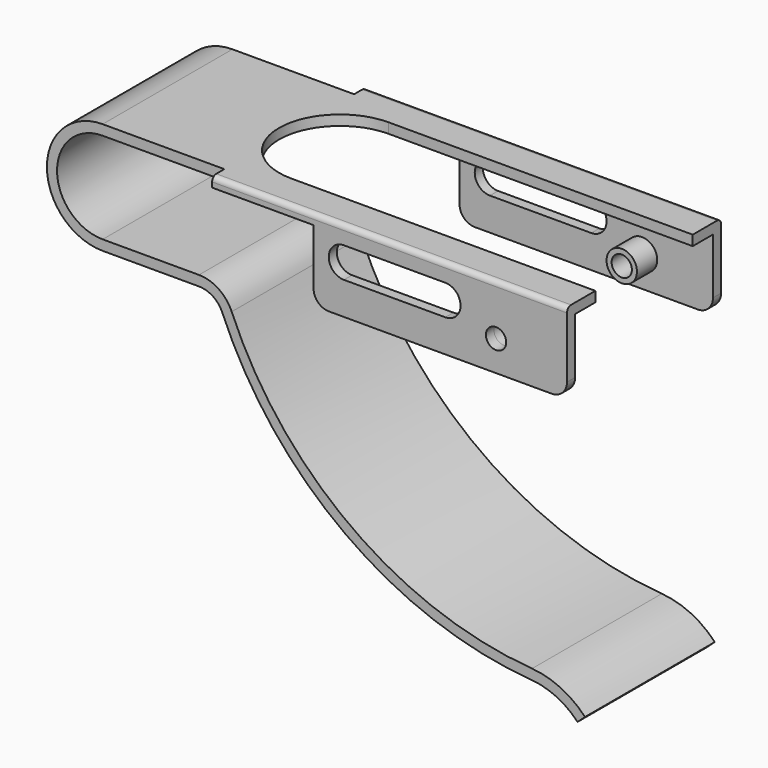
from build123d import *

# Parameters (mm, degrees)
F1_DEPTH  = 16
F2_W      = 70
F2_H      = 3
F3_DEPTH  = 2
F4_W      = 50
F4_H      = 14
F5_DEPTH  = 2
F6_R      = 1
F9_DEPTH  = 2
F11_DEPTH = 38.001
F13_D     = 4
F14_R     = 3
F14_R_2   = 2
F15_DEPTH = 5
F16_R     = 3


# Not quite as in the source:
# - a pattern or mirror of a feature is missing from the dataset's text; its kind, count and spacing are read off the source's solid


with BuildPart() as f1:
    # F0 (on Front) → F1 (new body)
    with BuildSketch(Plane.XZ):
        with BuildLine():
            Line((94, 11), (0, 11))
            ThreePointArc((0, 11), (-11, 0), (0, -11))
            Line((0, -11), (19, -11))
            ThreePointArc((19, -11), (21.7681124643, -11.8361612201), (23.6103896104, -14.064978646))
            ThreePointArc((23.6103896104, -14.064978646), (47.8977113224, -44.6078392712), (84.5520957277, -57.9942665386))
            ThreePointArc((84.5520957277, -57.9942665386), (89.5187953856, -59.3173941728), (93.6732506492, -62.3438233708))
            Line((93.6732506492, -62.3438233708), (95.1549842887, -61))
            ThreePointArc((95.1549842887, -61), (90.3976747979, -57.5207528796), (84.7034264019, -56))
            ThreePointArc((84.7034264019, -56), (49.0672193413, -42.9854179344), (25.4545454545, -13.2909701044))
            ThreePointArc((25.4545454545, -13.2909701044), (22.87535745, -10.1706257081), (19, -9))
            Line((19, -9), (0, -9))
            ThreePointArc((0, -9), (-9, 0), (0, 9))
            Line((0, 9), (94, 9))
            Line((94, 9), (94, 11))
        make_face()
    extrude(amount=F1_DEPTH)

    # F2 (on face) → F3 (join)
    with BuildSketch(Plane.XY.offset(11)):
        with Locations((59, -17.5)):
            Rectangle(F2_W, F2_H)
    extrude(amount=-F3_DEPTH)

    # F4 (on face) → F5 (join)
    with BuildSketch(Plane.XZ.offset(19)):
        with Locations((69, 2)):
            Rectangle(F4_W, F4_H)
    extrude(amount=-F5_DEPTH)

    # F6
    f6_edges = [f1.edges().sort_by_distance(p)[0] for p in [
        (59, -19, 11),
    ]]
    fillet(f6_edges, radius=F6_R)

    # F7: F1 across plane


with BuildPart() as f1_1:
    add(f1.part)
    add(f1.part.mirror(Plane.XZ))

    # F8 (on face) → F9 (cut)
    with BuildSketch(Plane.XY.offset(11)):
        with BuildLine():
            Line((94, 12), (34, 12))
            ThreePointArc((34, 12), (22, 0), (34, -12))
            Line((34, -12), (94, -12))
            Line((94, -12), (94, 12))
        make_face()
    extrude(amount=-F9_DEPTH, mode=Mode.SUBTRACT)

    # F10 (on face) → F11 (cut, through all)
    with BuildSketch(Plane.XZ.offset(19)):
        with BuildLine():
            ThreePointArc((50, 7.4429814443), (47, 4.4429814443), (50, 1.4429814443))
            Line((50, 1.4429814443), (70, 1.4429814443))
            ThreePointArc((70, 1.4429814443), (73, 4.4429814443), (70, 7.4429814443))
            Line((70, 7.4429814443), (50, 7.4429814443))
        make_face()
    extrude(amount=-F11_DEPTH, mode=Mode.SUBTRACT)

    # F13 (through all)
    with Locations(Plane.XZ.offset(19)):
        with Locations((80, 1)):
            Hole(F13_D / 2)

    # F14 (on face) → F15 (join)
    with BuildSketch(Plane(origin=(0, -17, 0), x_dir=(-1, 0, 0), z_dir=(0, 1, 0))):
        with Locations((-80, 1)):
            Circle(F14_R)
        with Locations((-80, 1)):
            Circle(F14_R_2, mode=Mode.SUBTRACT)
    f15 = extrude(amount=F15_DEPTH)

    # F15_copies: F15 across plane
    add(f15.mirror(Plane.ZX))

    # F16
    f16_edges = [f1_1.edges().sort_by_distance(p)[0] for p in [
        (94, 18, -5),
        (44, 18, -5),
        (94, -18, -5),
        (44, -18, -5),
    ]]
    fillet(f16_edges, radius=F16_R)


solid = f1_1.part
